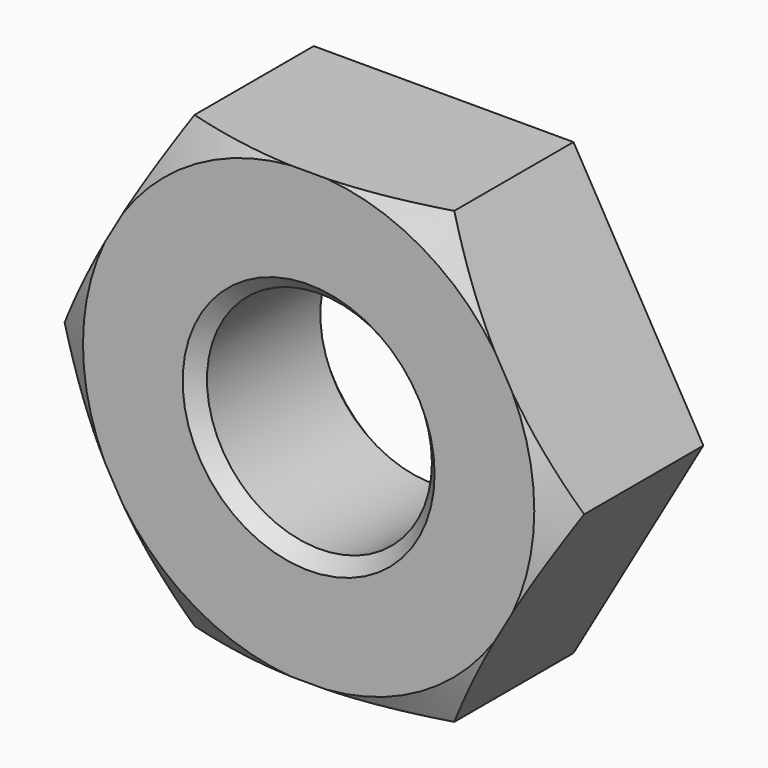
from build123d import *

# Parameters (mm, degrees)
F0_R     = 6.35
F1_DEPTH = 4.7625
F2_SIZE  = 0.762


# Not quite as in the source:
# - a feature names something its author has since deleted; it is built from what else it names


with BuildPart() as f1:
    # F0 (on Front) → F1 (new body, symmetric)
    with BuildSketch(Plane.XZ):
        Polygon((7.3323484187, 12.7), (-7.3323484187, 12.7), (-14.6646968374, 0), (-7.3323484187, -12.7), (7.3323484187, -12.7), (14.6646968374, 0), align=None)
        Circle(F0_R, mode=Mode.SUBTRACT)
    extrude(amount=F1_DEPTH, both=True)

    # F2
    f2_edges = [f1.edges().sort_by_distance(p)[0] for p in [
        (-6.35, -4.7625, 0),
        (-6.35, 4.7625, 0),
    ]]
    chamfer(f2_edges, length=F2_SIZE)

    # F4: sweep along a path in F4_path
    with BuildLine(Plane(origin=(7.112, -4.7625, 0), x_dir=(0, 0, -1), z_dir=(0, 1, 0))) as f4_path:
        CenterArc((0, 7.112), 7.112, 0, 360)
    # F3 (on Top) → F4 (sweep, cut)
    with BuildSketch(Plane.XY):
        Polygon((-14.8424788945, -5.049383917), (-12.7, -4.7852232567), (-14.8424788945, -3.5482624902), align=None)
    sweep(path=f4_path.line, mode=Mode.SUBTRACT)


solid = f1.part
